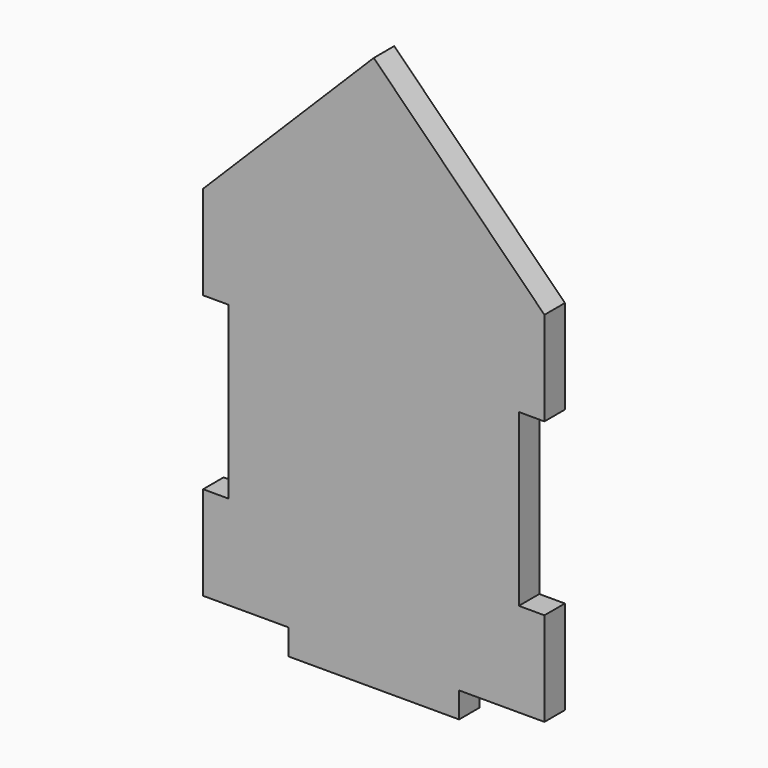
from build123d import *

# Parameters (mm, degrees)
F0_W     = 20
F0_H     = 40
F0_H_2   = 3
F1_DEPTH = 3


# Not quite as in the source:
# - a feature names something its author has since deleted; it is built from what else it names


with BuildPart() as f1:
    # F0 (on Front) → F1 (new body)
    with BuildSketch(Plane.XZ):
        Polygon((10, -21), (20, -21), (20, -10), (17, -10), (17, 10), (20, 10), (20, 21), (0, 41), (-20, 21), (-20, 10), (-17, 10), (-17, -10), (-20, -10), (-20, -21), (-10, -21), (-10, 19), (10, 19), align=None)
        with Locations((0, -1)):
            Rectangle(F0_W, F0_H)
        with Locations((0, -22.5)):
            Rectangle(F0_W, F0_H_2)
    extrude(amount=-F1_DEPTH)


solid = f1.part
